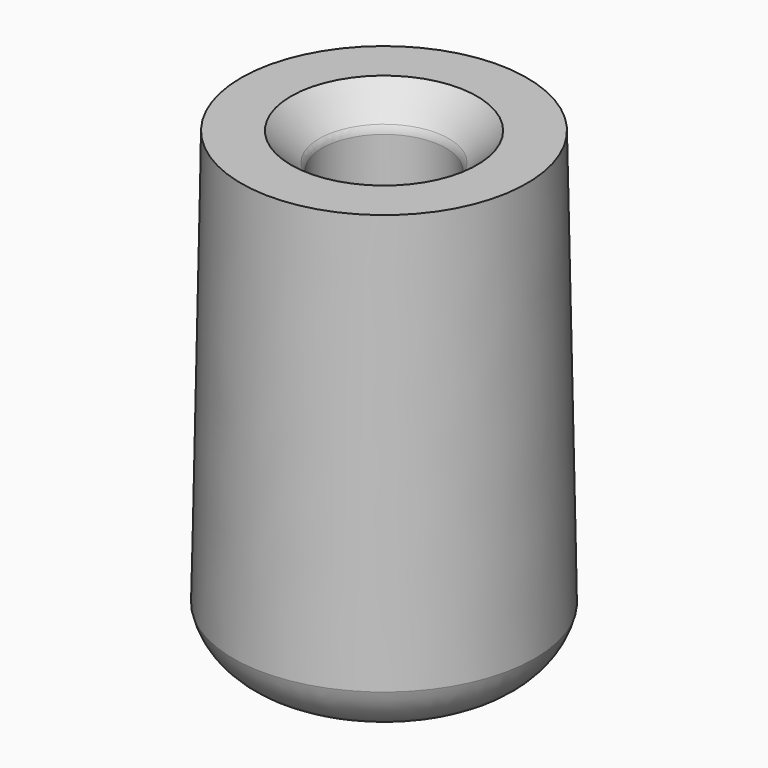
from build123d import *

# Parameters (mm, degrees)
F0_R     = 2.9
F1_DEPTH = 1
F5_SIZE  = 0.6
F6_R     = 0.2


# Not quite as in the source:
# - a fillet or chamfer that OpenCascade refuses, or shapes differently, is made with other operations: its cross-section is extruded or revolved along the edge and cut away or added


with BuildPart() as f1:
    # F0 (on Top) → F1 (new body)
    with BuildSketch(Plane.XY):
        Circle(F0_R)
    extrude(amount=F1_DEPTH)

    # F4: fillet of radius 1.3 on 1 edges, made by hand

    # F4_s1 → F4_t2 (revolve, cut)
    with BuildSketch(Plane.XZ):
        with BuildLine():
            ThreePointArc((2.9, 1), (2.4413147108, 0.2801960973), (1.6350889359, 0))
            Line((1.6350889359, 0), (2.9, 0))
            Line((2.9, 0), (2.9, 1))
        make_face()
    revolve(axis=Axis((0, 0, 0), (0, 0, 1)), mode=Mode.SUBTRACT)


with BuildPart() as f3:
    # F2 (on Front) → F3 (revolve)
    with BuildSketch(Plane.XZ):
        Polygon((-2.9, 1), (-1.19, 1), (-1.19, 9), (-2.75, 9), align=None)
    revolve(axis=Axis((0, 0, 5), (0, 0, -1)))

    # F5
    f5_edges = [f3.edges().sort_by_distance(p)[0] for p in [
        (1.19, 0, 9),
    ]]
    chamfer(f5_edges, length=F5_SIZE)

    # F6
    f6_edges = [f3.edges().sort_by_distance(p)[0] for p in [
        (1.19, 0, 8.4),
    ]]
    fillet(f6_edges, radius=F6_R)


solid = Compound([f1.part, f3.part])
